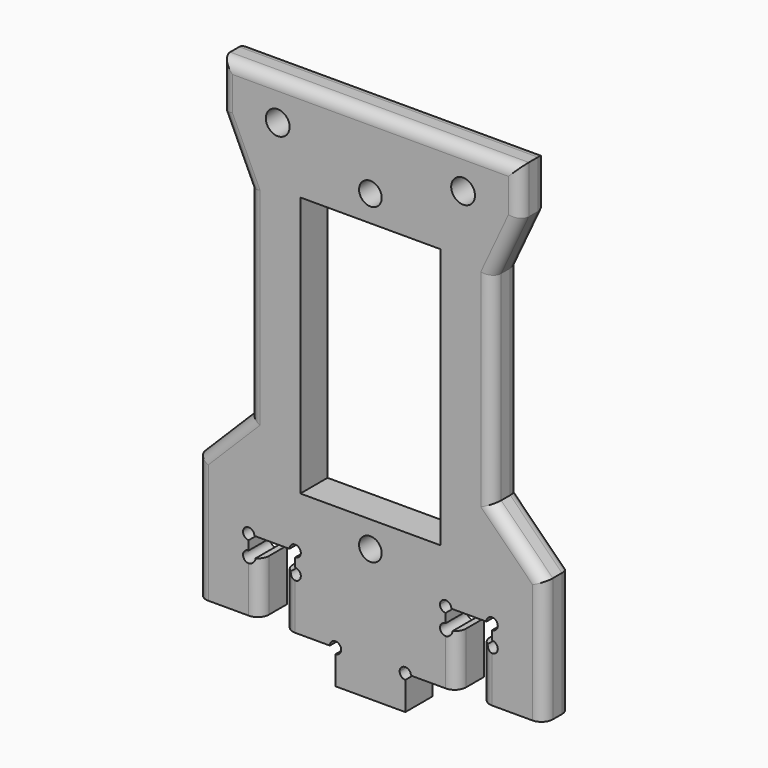
from build123d import *

# Parameters (mm, degrees)
F0_R     = 1.05
F0_R_2   = 1
F1_DEPTH = 3
F2_R     = 1


# Not quite as in the source:
# - a feature names something its author has since deleted; it is built from what else it names


with BuildPart() as f1:
    # F0 (on Front) → F1 (new body)
    with BuildSketch(Plane.XZ):
        with BuildLine():
            ThreePointArc((3.08, -22.97), (2.7264466094, -22.8235533906), (2.58, -22.47))
            Line((2.58, -22.47), (-2.58, -22.47))
            ThreePointArc((-2.58, -22.47), (-2.7264466094, -22.8235533906), (-3.08, -22.97))
            Line((-3.08, -22.97), (-3.08, -25.47))
            Line((-3.08, -25.47), (3.08, -25.47))
            Line((3.08, -25.47), (3.08, -22.97))
        make_face()
        Polygon((10.74, -6.94), (10.74, -11.5), (15.3, -11.5), align=None)
        Polygon((-15.3, -11.5), (-10.74, -11.5), (-10.74, -6.94), align=None)
        with BuildLine():
            Line((10.74, -11.5), (10.74, -15.61))
            ThreePointArc((10.74, -15.61), (11.24, -16.11), (10.74, -16.61))
            Line((10.74, -16.61), (10.74, -17.41))
            ThreePointArc((10.74, -17.41), (11.0935533906, -18.2635533906), (10.24, -17.91))
            Line((10.24, -17.91), (9.74, -17.91))
            Line((9.74, -17.91), (9.74, -22.47))
            Line((9.74, -22.47), (15.3, -22.47))
            Line((15.3, -22.47), (15.3, -11.5))
            Line((15.3, -11.5), (10.74, -11.5))
        make_face()
        with BuildLine():
            Line((-10.74, -15.61), (-10.74, -11.5))
            Line((-10.74, -11.5), (-15.3, -11.5))
            Line((-15.3, -11.5), (-15.3, -22.47))
            Line((-15.3, -22.47), (-9.74, -22.47))
            Line((-9.74, -22.47), (-9.74, -17.91))
            Line((-9.74, -17.91), (-10.24, -17.91))
            ThreePointArc((-10.24, -17.91), (-11.0935533906, -18.2635533906), (-10.74, -17.41))
            Line((-10.74, -17.41), (-10.74, -16.61))
            ThreePointArc((-10.74, -16.61), (-11.24, -16.11), (-10.74, -15.61))
        make_face()
        Polygon((6.18, -11.5), (10.74, -11.5), (10.74, -6.94), (10.74, 10.6763684678), (13.18, 15.9089653538), (13.18, 20.1089653538), (-13.18, 20.1089653538), (-13.18, 15.9089653538), (-10.74, 10.6763684678), (-10.74, -6.94), (-10.74, -11.5), (-6.18, -11.5), (-6.18, 11.5), (6.18, 11.5), align=None)
        with Locations((-8.18, 16.6589653538)):
            Circle(F0_R, mode=Mode.SUBTRACT)
        with Locations((0, 13.805)):
            Circle(F0_R_2, mode=Mode.SUBTRACT)
        with Locations((8.18, 16.6589653538)):
            Circle(F0_R, mode=Mode.SUBTRACT)
        with BuildLine():
            ThreePointArc((6.64, -16.61), (6.2864466094, -16.4635533906), (6.14, -16.11))
            Line((6.14, -16.11), (-6.14, -16.11))
            ThreePointArc((-6.14, -16.11), (-6.2864466094, -16.4635533906), (-6.64, -16.61))
            Line((-6.64, -16.61), (-6.64, -17.41))
            ThreePointArc((-6.64, -17.41), (-6.2864466094, -18.2635533906), (-7.14, -17.91))
            Line((-7.14, -17.91), (-7.64, -17.91))
            Line((-7.64, -17.91), (-7.64, -22.47))
            Line((-7.64, -22.47), (-3.58, -22.47))
            ThreePointArc((-3.58, -22.47), (-3.08, -21.97), (-2.58, -22.47))
            Line((-2.58, -22.47), (2.58, -22.47))
            ThreePointArc((2.58, -22.47), (3.08, -21.97), (3.58, -22.47))
            Line((3.58, -22.47), (7.64, -22.47))
            Line((7.64, -22.47), (7.64, -17.91))
            Line((7.64, -17.91), (7.14, -17.91))
            ThreePointArc((7.14, -17.91), (6.2864466094, -18.2635533906), (6.64, -17.41))
            Line((6.64, -17.41), (6.64, -16.61))
        make_face()
        with BuildLine():
            ThreePointArc((6.14, -16.11), (6.1501020514, -16.01), (6.18, -15.9140408206))
            Line((6.18, -15.9140408206), (6.18, -11.5))
            Line((6.18, -11.5), (-6.18, -11.5))
            Line((-6.18, -11.5), (-6.18, -15.9140408206))
            ThreePointArc((-6.18, -15.9140408206), (-6.1501020514, -16.01), (-6.14, -16.11))
            Line((-6.14, -16.11), (6.14, -16.11))
        make_face()
        with Locations((0, -13.805)):
            Circle(F0_R_2, mode=Mode.SUBTRACT)
        with BuildLine():
            Line((-6.18, -15.9140408206), (-6.18, -11.5))
            Line((-6.18, -11.5), (-10.74, -11.5))
            Line((-10.74, -11.5), (-10.74, -15.61))
            ThreePointArc((-10.74, -15.61), (-10.3864466094, -15.7564466094), (-10.24, -16.11))
            Line((-10.24, -16.11), (-7.14, -16.11))
            ThreePointArc((-7.14, -16.11), (-6.74, -15.6201020514), (-6.18, -15.9140408206))
        make_face()
        with BuildLine():
            Line((7.14, -16.11), (10.24, -16.11))
            ThreePointArc((10.24, -16.11), (10.3864466094, -15.7564466094), (10.74, -15.61))
            Line((10.74, -15.61), (10.74, -11.5))
            Line((10.74, -11.5), (6.18, -11.5))
            Line((6.18, -11.5), (6.18, -15.9140408206))
            ThreePointArc((6.18, -15.9140408206), (6.74, -15.6201020514), (7.14, -16.11))
        make_face()
    extrude(amount=F1_DEPTH)

    # F2
    f2_edges = [f1.edges().sort_by_distance(p)[0] for p in [
        (0, -3, 20.108965),
        (-13.18, -3, 18.008965),
        (-11.96, -3, 13.292667),
        (-10.74, -3, 1.868184),
        (-13.02, -3, -9.22),
        (-15.3, -3, -16.985),
        (15.3, -3, -16.985),
        (13.02, -3, -9.22),
        (10.74, -3, 1.868184),
        (11.96, -3, 13.292667),
        (13.18, -3, 18.008965),
        (7.64, -3, -20.19),
        (9.74, -3, -20.19),
        (-7.64, -3, -20.19),
        (-9.74, -3, -20.19),
        (0, 0, 20.108965),
        (13.18, 0, 18.008965),
        (11.96, 0, 13.292667),
        (-13.18, 0, 18.008965),
        (-11.96, 0, 13.292667),
        (-10.74, 0, 1.868184),
        (-13.02, 0, -9.22),
        (-15.3, 0, -16.985),
        (15.3, 0, -16.985),
        (13.02, 0, -9.22),
        (10.74, 0, 1.868184),
    ]]
    fillet(f2_edges, radius=F2_R)


solid = f1.part
